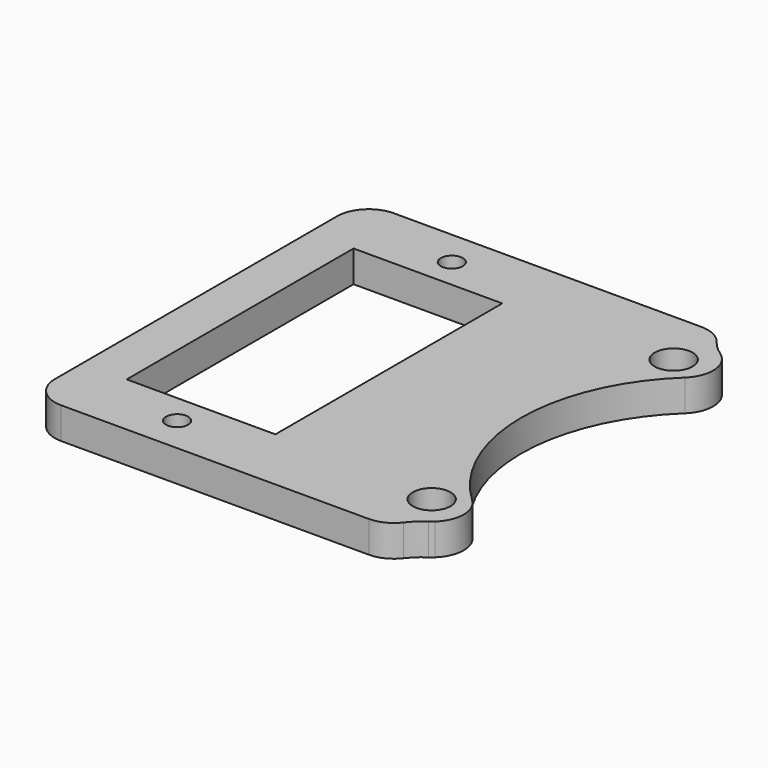
from build123d import *

# Parameters (mm, degrees)
F0_R        = 0.875
F0_W        = 24.8
F0_H        = 1.5
F0_R_2      = 1.5
F0_W_2      = 3.5
F1_DEPTH    = 2.5
F2_T1_DEPTH = 2.5
F3_R        = 2.5


# Not quite as in the source:
# - a fillet or chamfer that OpenCascade refuses, or shapes differently, is made with other operations: its cross-section is extruded or revolved along the edge and cut away or added


with BuildPart() as f1:
    # F0 (on Top) → F1 (new body)
    with BuildSketch(Plane.XY):
        with BuildLine():
            Line((-36.8, -15), (-12, -15))
            ThreePointArc((-12, -15), (-14.1213203436, -14.1213203436), (-15, -12))
            Line((-15, -12), (-15, 12))
            ThreePointArc((-15, 12), (-14.1213203436, 14.1213203436), (-12, 15))
            Line((-12, 15), (-36.8, 15))
            Line((-36.8, 15), (-36.8, 11.25))
            Line((-36.8, 11.25), (-25, 11.25))
            Line((-25, 11.25), (-25, -11.25))
            Line((-25, -11.25), (-36.8, -11.25))
            Line((-36.8, -11.25), (-36.8, -15))
        make_face()
        with Locations((-30.9, -13.625)):
            Circle(F0_R, mode=Mode.SUBTRACT)
        with Locations((-30.9, 13.625)):
            Circle(F0_R, mode=Mode.SUBTRACT)
        with Locations((-24.4, -15.75)):
            Rectangle(F0_W, F0_H)
        with BuildLine():
            ThreePointArc((-15, -12), (-14.1213203436, -14.1213203436), (-12, -15))
            ThreePointArc((-12, -15), (-9.6452475907, -13.8588009821), (-9.0819892727, -11.3034273939))
            ThreePointArc((-9.0819892727, -11.3034273939), (-14.5, 0), (-9.0819892727, 11.3034273939))
            ThreePointArc((-9.0819892727, 11.3034273939), (-9.6452475907, 13.8588009821), (-12, 15))
            ThreePointArc((-12, 15), (-14.1213203436, 14.1213203436), (-15, 12))
            Line((-15, 12), (-15, -12))
        make_face()
        with Locations((-12, -12)):
            Circle(F0_R_2, mode=Mode.SUBTRACT)
        with Locations((-12, 12)):
            Circle(F0_R_2, mode=Mode.SUBTRACT)
        with Locations((-38.55, -15.75)):
            Rectangle(F0_W_2, F0_H)
        Polygon((-40.3, -15), (-36.8, -15), (-36.8, -11.25), (-36.8, 11.25), (-36.8, 15), (-40.3, 15), align=None)
        with Locations((-24.4, 15.75)):
            Rectangle(F0_W, F0_H)
        with Locations((-38.55, 15.75)):
            Rectangle(F0_W_2, F0_H)
    extrude(amount=F1_DEPTH)

    # F2: fillet of radius 5 on 2 edges, made by hand

    # F2_s2 → F2_t1 (join)
    with BuildSketch(Plane.XY):
        with BuildLine():
            ThreePointArc((-10.2955137321, 14.46875), (-11.284865017, 15.3693232041), (-12, 16.5))
            Line((-12, 16.5), (-12, 15))
            ThreePointArc((-12, 15), (-11.1073214464, 14.8641098093), (-10.2955137321, 14.46875))
        make_face()
        with BuildLine():
            ThreePointArc((-12, -16.5), (-11.284865017, -15.3693232041), (-10.2955137321, -14.46875))
            ThreePointArc((-10.2955137321, -14.46875), (-11.1073214464, -14.8641098093), (-12, -15))
            Line((-12, -15), (-12, -16.5))
        make_face()
    extrude(amount=F2_T1_DEPTH)

    # F3
    f3_edges = [f1.edges().sort_by_distance(p)[0] for p in [
        (-12, 16.5, 1.25),
        (-12, -16.5, 1.25),
        (-9.081989, 11.303427, 1.25),
        (-9.081989, -11.303427, 1.25),
        (-40.3, 16.5, 1.25),
        (-40.3, -16.5, 1.25),
    ]]
    fillet(f3_edges, radius=F3_R)


solid = f1.part
